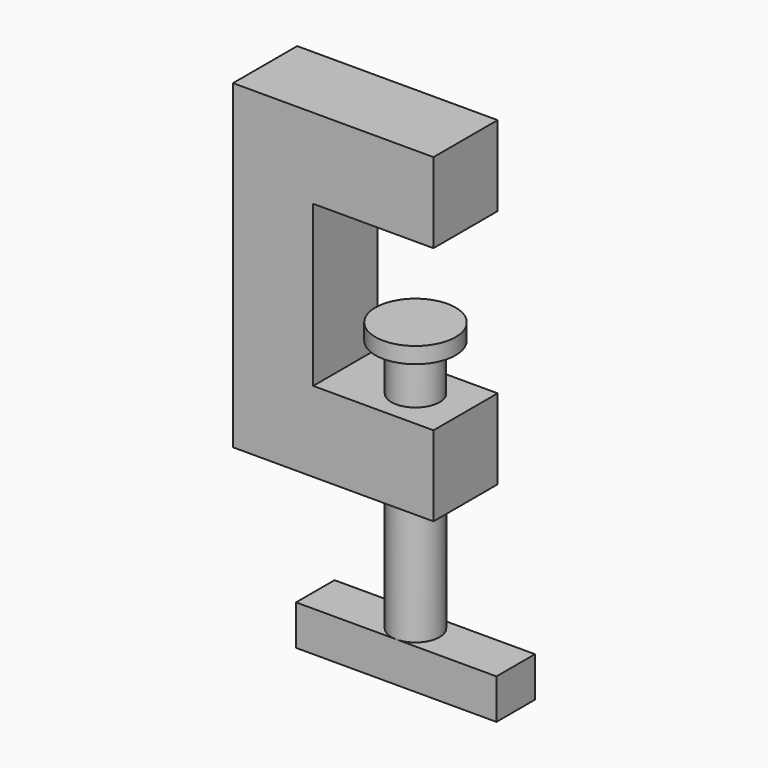
from build123d import *

# Parameters (mm, degrees)
F0_W     = 15
F0_H     = 10
F1_DEPTH = 10
F2_R     = 3
F3_DEPTH = 15.8
F5_DEPTH = 5
F6_R     = 5
F6_R_2   = 3
F7_DEPTH = 2


with BuildPart() as f1:
    # F0 (on Front) → F1 (new body)
    with BuildSketch(Plane.XZ):
        Polygon((-10, 0), (0, 0), (0, 10), (0, 30), (0, 40), (-10, 40), align=None)
        with Locations((7.5, 5)):
            Rectangle(F0_W, F0_H)
        with Locations((7.5, 35)):
            Rectangle(F0_W, F0_H)
    extrude(amount=F1_DEPTH)

    # F2 (on face) → F3 (join, symmetric)
    with BuildSketch(Plane(origin=(0, 0, 0), x_dir=(1, 0, 0), z_dir=(0, 0, -1))):
        with Locations((8.7596364319, 5)):
            Circle(F2_R)
    extrude(amount=F3_DEPTH, both=True)

    # F4 (on face) → F5 (join)
    with BuildSketch(Plane(origin=(0, 0, -15.8), x_dir=(1, 0, 0), z_dir=(0, 0, -1))):
        with BuildLine():
            Line((-3.7403635681, 2), (8.7596364319, 2))
            ThreePointArc((8.7596364319, 2), (5.7596364319, 5), (8.7596364319, 8))
            Line((8.7596364319, 8), (-3.7403635681, 8))
            Line((-3.7403635681, 8), (-3.7403635681, 2))
        make_face()
        with BuildLine():
            Line((8.7596364319, 2), (21.2596364319, 2))
            Line((21.2596364319, 2), (21.2596364319, 8))
            Line((21.2596364319, 8), (8.7596364319, 8))
            ThreePointArc((8.7596364319, 8), (10.8809567755, 7.1213203436), (11.7596364319, 5))
            ThreePointArc((11.7596364319, 5), (10.8809567755, 2.8786796564), (8.7596364319, 2))
        make_face()
        with BuildLine():
            ThreePointArc((8.7596364319, 8), (5.7596364319, 5), (8.7596364319, 2))
            ThreePointArc((8.7596364319, 2), (10.8809567755, 2.8786796564), (11.7596364319, 5))
            ThreePointArc((11.7596364319, 5), (10.8809567755, 7.1213203436), (8.7596364319, 8))
        make_face()
    extrude(amount=F5_DEPTH)

    # F6 (on face) → F7 (join)
    with BuildSketch(Plane.XY.offset(15.8)):
        with Locations((8.7596364319, -5)):
            Circle(F6_R)
        with Locations((8.7596364319, -5)):
            Circle(F6_R_2, mode=Mode.SUBTRACT)
        with Locations((8.7596364319, -5)):
            Circle(F6_R_2)
    extrude(amount=F7_DEPTH)


solid = f1.part
